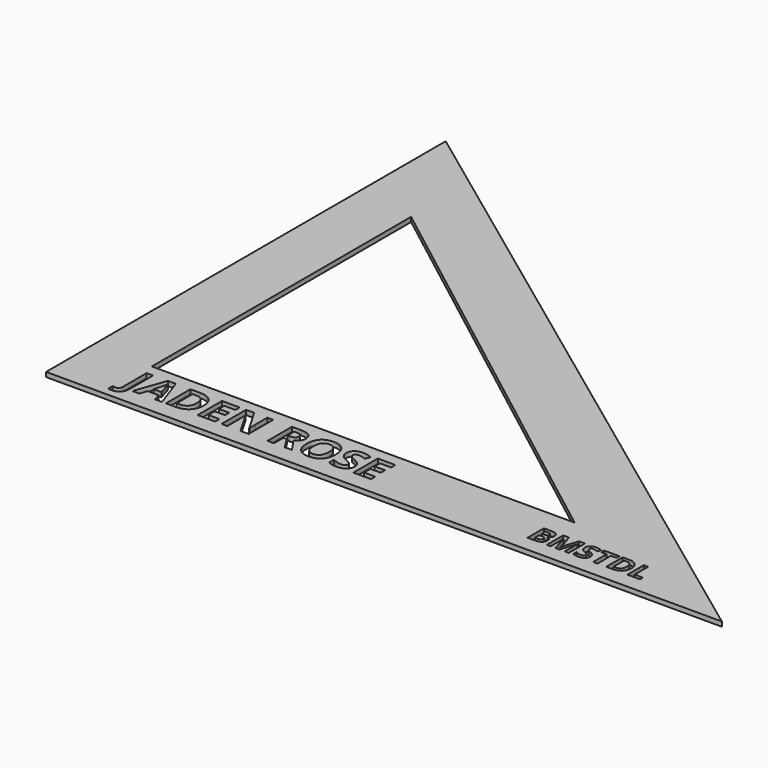
from build123d import *

# Parameters (mm, degrees)
F1_DEPTH       = 2
F2_SCALE       = 0.75
F3_TEXT_SIZE   = 13.8751121122
F3_TEXT_SIZE_2 = 9.2873349786
F4_DEPTH       = 1.501


# Not quite as in the source:
# - Text() gives the source's letters only with a copy of the font that has no kerning and outlines rounded to 1/6400 em; it was checked with that copy


with BuildPart() as f1:
    # F0 (on Top) → F1 (new body)
    with BuildSketch(Plane.XY):
        Polygon((-110.3935540405, 109.5033976257), (-110.3935540405, -106.3966023743), (181.7064459595, -106.3966023743), align=None)
        Polygon((-84.9935540405, -80.9966023743), (-84.9935540405, 59.0477188125), (97.7188157638, -80.9966023743), align=None, mode=Mode.SUBTRACT)
    extrude(amount=F1_DEPTH)


with BuildPart() as f1_1:
    # F2: moved
    add(f1.part.scale(F2_SCALE))

    # F3 (on face) → F4 (cut, through all)
    with BuildSketch(Plane.XY.offset(1.5)):
        with Locations((-63.7451655304, -74.3297189474)):
            Text('JADEN ROSE', F3_TEXT_SIZE, font='Open Sans', font_style=FontStyle.BOLD, text_align=(TextAlign.LEFT, TextAlign.BOTTOM))
        with Locations((68.3347433805, -74.6641978621)):
            Text('BMSTDL', F3_TEXT_SIZE_2, font='Open Sans', font_style=FontStyle.BOLD, text_align=(TextAlign.LEFT, TextAlign.BOTTOM))
    extrude(amount=-F4_DEPTH, mode=Mode.SUBTRACT)


solid = f1_1.part
